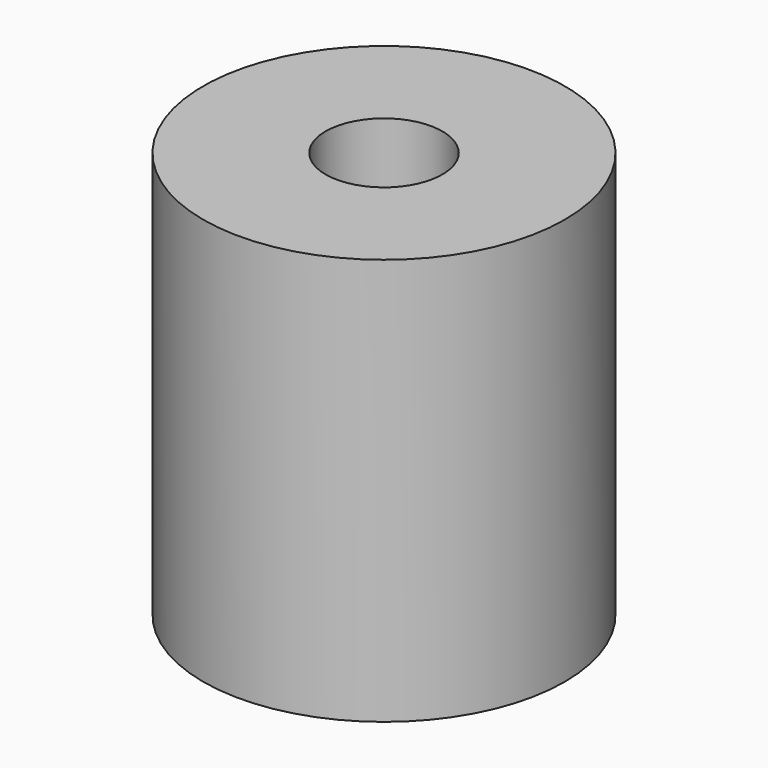
from build123d import *

# Parameters (mm, degrees)
F0_R     = 12.7
F1_DEPTH = 28.575
F3_D     = 8.2042


# Not quite as in the source:
# - a feature names something its author has since deleted; it is built from what else it names


with BuildPart() as f1:
    # F0 (on Top) → F1 (new body)
    with BuildSketch(Plane.XY):
        Circle(F0_R)
    extrude(amount=F1_DEPTH)

    # F3 (through all)
    with Locations(Plane.XY.offset(28.575)):
        with Locations((0, 0)):
            Hole(F3_D / 2)


solid = f1.part
